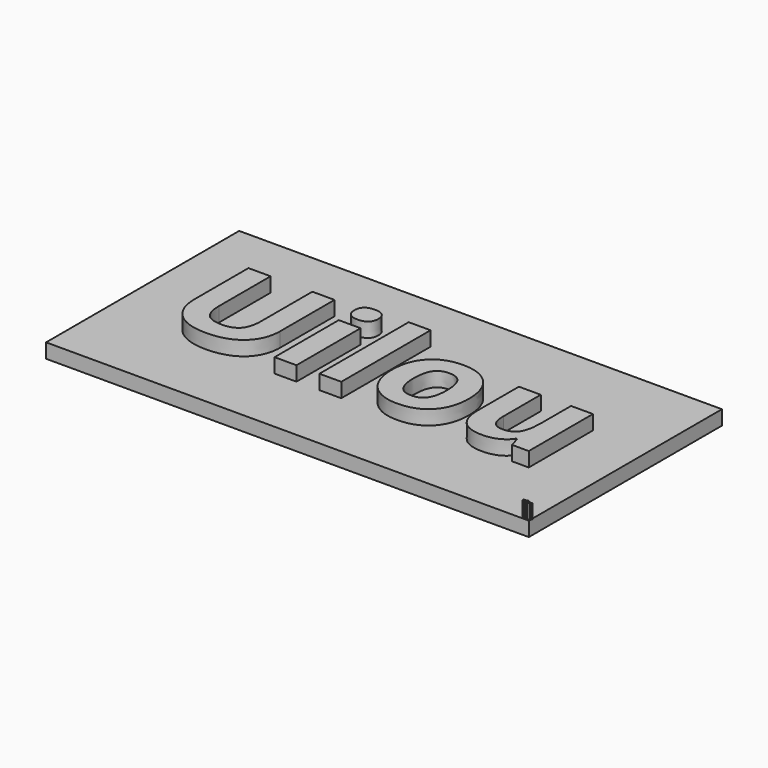
from build123d import *

# Parameters (mm, degrees)
F1_DEPTH       = 3
F3_TEXT_SIZE   = 0.7606370335
F3_TEXT_SIZE_2 = 30.4254813406
F4_DEPTH       = 3


# Not quite as in the source:
# - Text() gives the source's letters only with a copy of the font that has no kerning and outlines rounded to 1/6400 em; it was checked with that copy


with BuildPart() as f1:
    # F0 (on Top) → F1 (new body)
    with BuildSketch(Plane.XY):
        Polygon((-100, 0), (0, 0), (0, 50), (-50, 50), (-67.3830643688, 50), (-100, 50), align=None)
    extrude(amount=F1_DEPTH)

    # F3 (on face) → F4 (join)
    with BuildSketch(Plane.XY.offset(3)):
        with Locations((-1.7606959694, 0.3123363136)):
            Text('Uilou', F3_TEXT_SIZE, font='Open Sans', font_style=FontStyle.BOLD, text_align=(TextAlign.LEFT, TextAlign.BOTTOM))
        with Locations((-89.6713957191, 14.5369875076)):
            Text('Uilou', F3_TEXT_SIZE_2, font='Open Sans', font_style=FontStyle.BOLD, text_align=(TextAlign.LEFT, TextAlign.BOTTOM))
    extrude(amount=F4_DEPTH)


solid = f1.part
